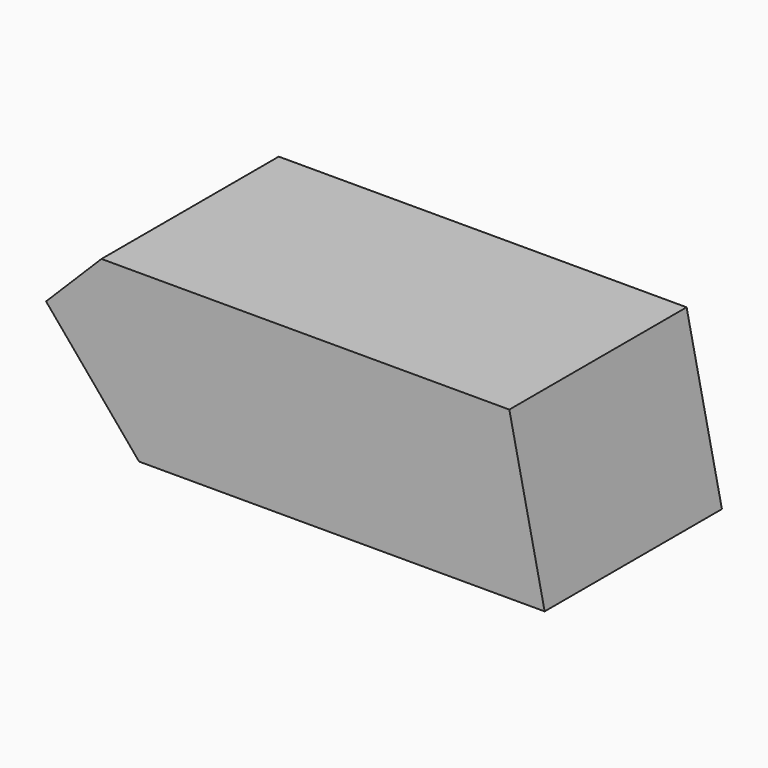
from build123d import *

# Parameters (mm, degrees)
F0_W     = 114.3
F0_H     = 50.8
F1_DEPTH = 38.1
F2_SIZE2 = 21.3131306319
F2_SIZE  = 25.4
F3_SIZE  = 12.69999
F4_SIZE2 = 8.098395
F4_SIZE  = 38.09999


# Not quite as in the source:
# - a fillet or chamfer is up to 0.001 mm smaller than in the source, because OpenCascade refuses the exact size


with BuildPart() as f1:
    # F0 (on Top) → F1 (new body)
    with BuildSketch(Plane.XY):
        with Locations((4.716448799, -1.0087825358)):
            Rectangle(F0_W, F0_H)
    extrude(amount=F1_DEPTH)

    # F2
    f2_edges = [f1.edges().sort_by_distance(p)[0] for p in [
        (-52.433551, -1.008783, 0),
    ]]
    f2_side = f1.faces().sort_by_distance((-52.433551, -1.008783, 19.05))[0]
    chamfer(f2_edges, length=F2_SIZE, length2=F2_SIZE2, reference=f2_side)

    # F3 (size 12.7 in the source; OpenCascade refuses exactly that, so slightly less here)
    f3_edges = [f1.edges().sort_by_distance(p)[0] for p in [
        (-52.433551, -1.008783, 38.1),
    ]]
    chamfer(f3_edges, length=F3_SIZE)

    # F4 (size 38.1 and 8.0984049996 in the source; OpenCascade refuses exactly that, so slightly less here)
    f4_edges = [f1.edges().sort_by_distance(p)[0] for p in [
        (61.866449, -1.008783, 38.1),
    ]]
    f4_side = f1.faces().sort_by_distance((61.866449, -1.008783, 19.05))[0]
    chamfer(f4_edges, length=F4_SIZE, length2=F4_SIZE2, reference=f4_side)


solid = f1.part
